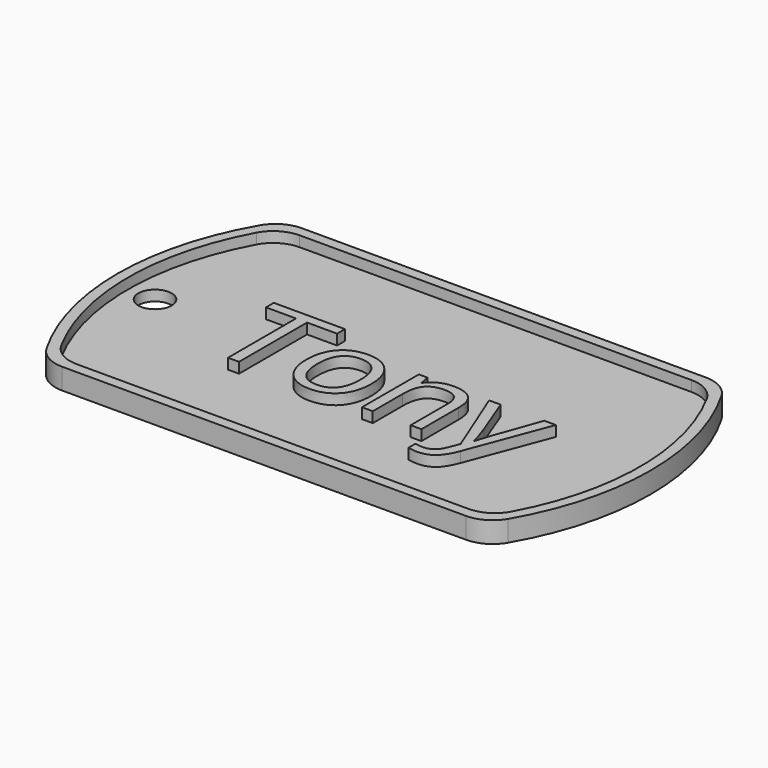
from build123d import *

# Parameters (mm, degrees)
F1_DEPTH     = 1
F3_DEPTH     = 1
F4_R         = 1.5875
F5_DEPTH     = 1
F6_TEXT_SIZE = 12.6620185458
F7_DEPTH     = 1


# Not quite as in the source:
# - Text() gives the source's letters only with a copy of the font that has no kerning and outlines rounded to 1/6400 em; it was checked with that copy


with BuildPart() as f1:
    # F0 (on Top) → F1 (new body)
    with BuildSketch(Plane.XY):
        with BuildLine():
            ThreePointArc((-19.2474145991, 14.2875), (-20.8349145991, 13.862130657), (-21.9970452561, 12.7))
            ThreePointArc((-21.9970452561, 12.7), (-25.4, 0), (-21.9970452561, -12.7))
            ThreePointArc((-21.9970452561, -12.7), (-20.8349145991, -13.862130657), (-19.2474145991, -14.2875))
            Line((-19.2474145991, -14.2875), (19.2474145991, -14.2875))
            ThreePointArc((19.2474145991, -14.2875), (20.8349145991, -13.862130657), (21.9970452561, -12.7))
            ThreePointArc((21.9970452561, -12.7), (25.4, 0), (21.9970452561, 12.7))
            ThreePointArc((21.9970452561, 12.7), (20.8349145991, 13.862130657), (19.2474145991, 14.2875))
            Line((19.2474145991, 14.2875), (-19.2474145991, 14.2875))
        make_face()
    extrude(amount=F1_DEPTH)

    # F2 (on face) → F3 (join)
    with BuildSketch(Plane.XY.offset(1)):
        with BuildLine():
            Line((19.2474145991, 14.2875), (-19.2474145991, 14.2875))
            ThreePointArc((-19.2474145991, 14.2875), (-20.8349145991, 13.862130657), (-21.9970452561, 12.7))
            ThreePointArc((-21.9970452561, 12.7), (-25.4, 0), (-21.9970452561, -12.7))
            ThreePointArc((-21.9970452561, -12.7), (-20.8349145991, -13.862130657), (-19.2474145991, -14.2875))
            Line((-19.2474145991, -14.2875), (19.2474145991, -14.2875))
            ThreePointArc((19.2474145991, -14.2875), (20.8349145991, -13.862130657), (21.9970452561, -12.7))
            ThreePointArc((21.9970452561, -12.7), (25.4, 0), (21.9970452561, 12.7))
            ThreePointArc((21.9970452561, 12.7), (20.8349145991, 13.862130657), (19.2474145991, 14.2875))
        make_face()
        with BuildLine():
            ThreePointArc((-21.4526124879, 11.6252061249), (-20.2856017842, 12.8404540819), (-18.6611352482, 13.2875))
            Line((-18.6611352482, 13.2875), (18.6611352482, 13.2875))
            ThreePointArc((18.6611352482, 13.2875), (20.2856017842, 12.8404540819), (21.4526124879, 11.6252061249))
            ThreePointArc((21.4526124879, 11.6252061249), (24.4, 0), (21.4526124879, -11.6252061249))
            ThreePointArc((21.4526124879, -11.6252061249), (20.2856017842, -12.8404540819), (18.6611352482, -13.2875))
            Line((18.6611352482, -13.2875), (-18.6611352482, -13.2875))
            ThreePointArc((-18.6611352482, -13.2875), (-20.2856017842, -12.8404540819), (-21.4526124879, -11.6252061249))
            ThreePointArc((-21.4526124879, -11.6252061249), (-24.4, 0), (-21.4526124879, 11.6252061249))
        make_face(mode=Mode.SUBTRACT)
    extrude(amount=F3_DEPTH)

    # F4 (on face) → F5 (cut)
    with BuildSketch(Plane.XY.offset(1)):
        with Locations((-21.821282804, 0)):
            Circle(F4_R)
    extrude(amount=-F5_DEPTH, mode=Mode.SUBTRACT)

    # F6 (on face) → F7 (join)
    with BuildSketch(Plane.XY.offset(1)):
        with Locations((-13.4827960283, -5.4483164568)):
            Text('Tony', F6_TEXT_SIZE, font='Open Sans', text_align=(TextAlign.LEFT, TextAlign.BOTTOM))
    extrude(amount=F7_DEPTH)


solid = f1.part
